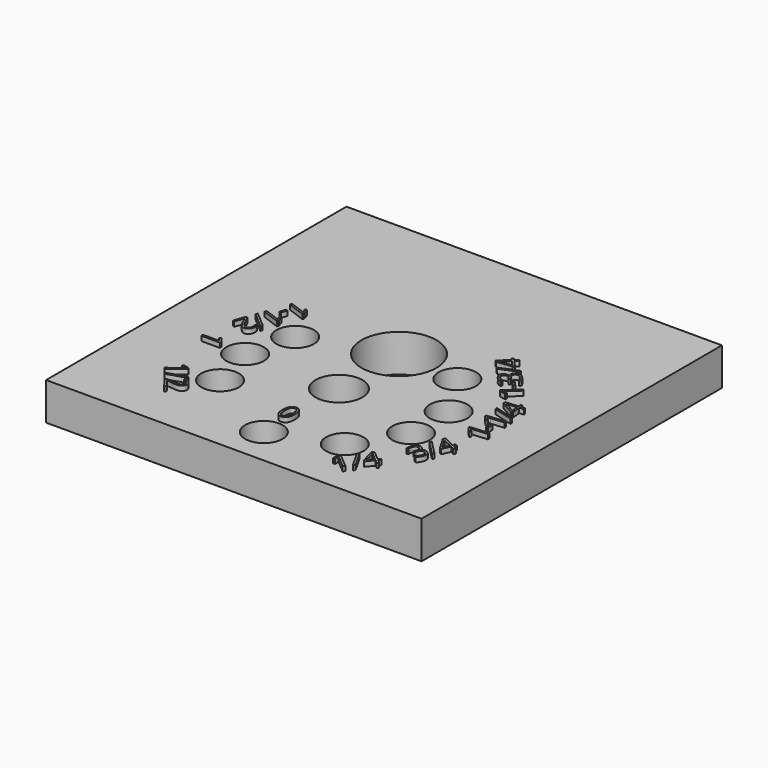
from build123d import *

# Parameters (mm, degrees)
F0_W         = 127
F0_H         = 127
F1_DEPTH     = 12.7
F3_D         = 12.7
F4_D         = 25.4
F5_D         = 15.875
F6_TEXT_SIZE = 8.8194444444
F7_DEPTH     = 1.5875


# Not quite as in the source:
# - Text() gives the source's letters only with a copy of the font that has no kerning and outlines rounded to 1/6400 em; it was checked with that copy


with BuildPart() as f1:
    # F0 (on Top) → F1 (new body)
    with BuildSketch(Plane.XY):
        with Locations((-12.053700164, 26.5172352473)):
            Rectangle(F0_W, F0_H)
    extrude(amount=F1_DEPTH)

    # F3 (through all)
    with Locations(Plane.XY.offset(12.7)):
        with Locations((-12.053700164, -24.2827647527), (-39.561900164, -8.4077647527), (-43.803700164, 7.4672352473), (-39.561900164, 23.3422352473), (8.952099836, 31.2670352473), (18.680299836, 15.4174352473), (18.680299836, -0.4829647527), (8.952099836, -16.3325647527)):
            Hole(F3_D / 2)

    # F4 (through all)
    with Locations(Plane.XY.offset(12.7)):
        with Locations((-12.053700164, 32.8672352473)):
            Hole(F4_D / 2)

    # F5 (through all)
    with Locations(Plane.XY.offset(12.7)):
        with Locations((-12.053700164, 7.4672352473)):
            Hole(F5_D / 2)

    # F6 (on face) → F7 (join)
    with BuildSketch(Plane.XY.offset(12.7)):
        with Locations(Location((16.733091967, -30.656932836), (0, 0, 50))):
            Text('1/4', F6_TEXT_SIZE, font='Open Sans', text_align=(TextAlign.LEFT, TextAlign.BOTTOM))
        with Locations(Location((30.15664526, -13.3077703641), (0, 0, 65))):
            Text('3/4', F6_TEXT_SIZE, font='Open Sans', text_align=(TextAlign.LEFT, TextAlign.BOTTOM))
        with Locations(Location((37.0237371751, 7.0510663257), (0, 0, 95))):
            Text('1-1/4', F6_TEXT_SIZE, font='Open Sans', text_align=(TextAlign.LEFT, TextAlign.BOTTOM))
        with Locations(Location((30.2795176478, 32.921110853), (0, 0, 132.2242617066))):
            Text('1-3/4', F6_TEXT_SIZE, font='Open Sans', text_align=(TextAlign.LEFT, TextAlign.BOTTOM))
        with Locations((-14.6981179714, -16.7697133332)):
            Text('0', F6_TEXT_SIZE, font='Open Sans', text_align=(TextAlign.LEFT, TextAlign.BOTTOM))
        with Locations(Location((-55.0274526857, -12.4214619382), (0, 0, -52.0974520401))):
            Text('1/2', F6_TEXT_SIZE, font='Open Sans', text_align=(TextAlign.LEFT, TextAlign.BOTTOM))
        with Locations(Location((-57.467239322, 9.1050690393), (0, 0, -90))):
            Text('1', F6_TEXT_SIZE, font='Open Sans', text_align=(TextAlign.LEFT, TextAlign.BOTTOM))
        with Locations(Location((-49.2987896949, 37.502550942), (0, 0, -110))):
            Text('1-1/2', F6_TEXT_SIZE, font='Open Sans', text_align=(TextAlign.LEFT, TextAlign.BOTTOM))
    extrude(amount=F7_DEPTH)


solid = f1.part
